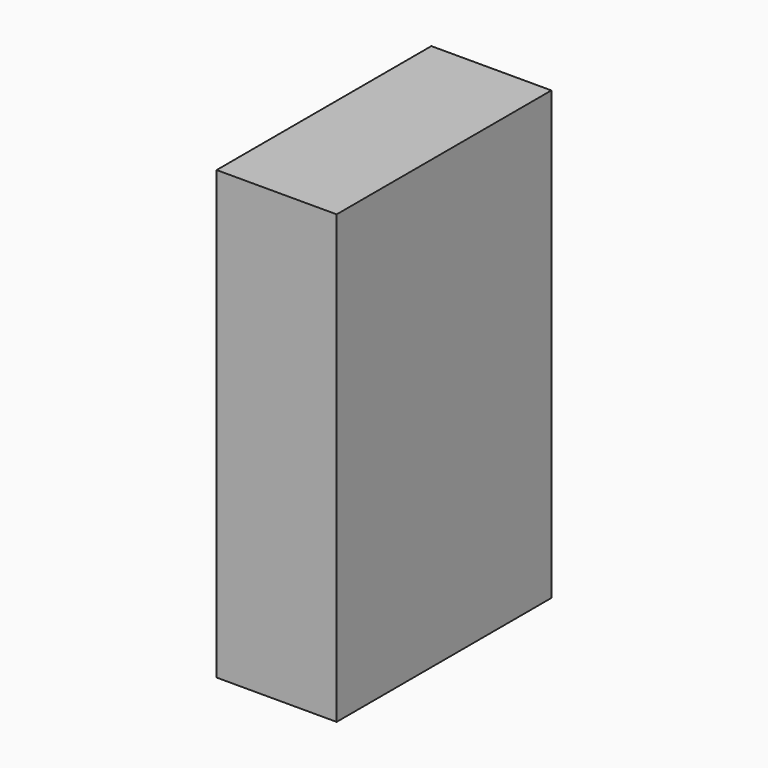
from build123d import *

# Parameters (mm, degrees)
F0_W     = 61.4049248397
F0_H     = 137.3135596514
F1_DEPTH = 228.6
F2_T     = -2.54
F7_R     = 5.08


# Not quite as in the source:
# - the program builds the solid bodies; features that only make, move or delete a surface that nothing else refers to are left out


with BuildPart() as f1:
    # F0 (on Top) → F1 (new body)
    with BuildSketch(Plane.XY):
        with Locations((30.7024624199, 68.6567798257)):
            Rectangle(F0_W, F0_H)
    extrude(amount=F1_DEPTH)

    # F2
    f2_openings = [f1.faces().sort_by_distance(p)[0] for p in [
        (0, 68.65678, 114.3),
    ]]
    offset(amount=F2_T, openings=f2_openings)

    # F7
    f7_edges = [f1.edges().sort_by_distance(p)[0] for p in [
        (58.864925, 134.77356, 114.3),
        (58.864925, 68.65678, 2.54),
        (58.864925, 2.54, 114.3),
        (58.864925, 68.65678, 226.06),
    ]]
    fillet(f7_edges, radius=F7_R)


solid = f1.part
